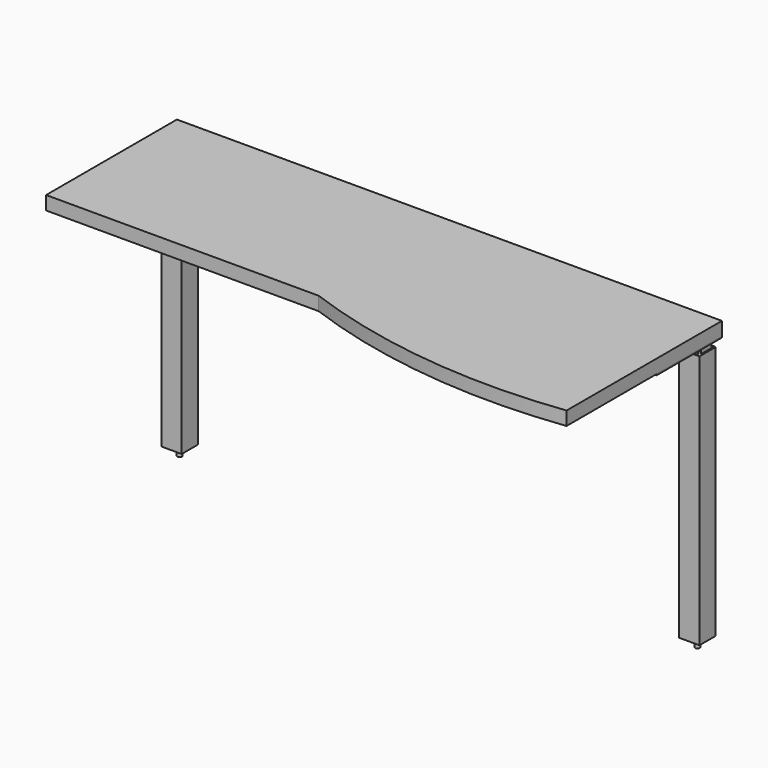
from build123d import *

# Parameters (mm, degrees)
F1_DEPTH = 38.1
F2_R     = 3.175
F2_W     = 57.0786401749
F2_H     = 56.9417057037
F2_R_2   = 6.35
F3_DEPTH = 3.175
F4_DEPTH = 685.8
F5_START = 25.4
F5_DEPTH = 25.4
F6_START = 25.4
F6_DEPTH = 711.2
F7_START = 6.35
F7_DEPTH = 755.65


with BuildPart() as f1:
    # F0 (on Top) → F1 (new body)
    with BuildSketch(Plane.XY):
        with BuildLine():
            Line((762, -250.8953552246), (762, 0))
            Line((762, 0), (762, 228.6))
            Line((762, 228.6), (0, 228.6))
            Line((0, 228.6), (-762, 228.6))
            Line((-762, 228.6), (-762, 0))
            Line((-762, 0), (-762, -228.6))
            Line((-762, -228.6), (0, -228.6))
            ThreePointArc((0, -228.6), (375.8490807179, -317.246080689), (762, -314.3953552246))
            Line((762, -314.3953552246), (762, -250.8953552246))
        make_face()
    extrude(amount=-F1_DEPTH)


with BuildPart() as f3:
    # F2 (on face) → F3 (new body)
    with BuildSketch(Plane(origin=(0, 0, -38.1), x_dir=(1, 0, 0), z_dir=(0, 0, -1))):
        Polygon((-762, -152.4), (-762, -228.6), (-685.8, -228.6), (-533.4, -228.6), (-533.4, -203.2), (-685.8, -203.2), (-685.8, -152.4), (-736.6, -152.4), (-736.6, 0), (-762, 0), align=None)
        with Locations((-647.7, -215.9)):
            Circle(F2_R, mode=Mode.SUBTRACT)
        with Locations((-609.6, -215.9)):
            Circle(F2_R, mode=Mode.SUBTRACT)
        with Locations((-723.9, -190.5)):
            Rectangle(F2_W, F2_H, mode=Mode.SUBTRACT)
        with Locations((-571.5, -215.9)):
            Circle(F2_R, mode=Mode.SUBTRACT)
        with Locations((-749.3, -114.3)):
            Circle(F2_R, mode=Mode.SUBTRACT)
        with Locations((-749.3, -76.2)):
            Circle(F2_R, mode=Mode.SUBTRACT)
        with Locations((-749.3, -38.1)):
            Circle(F2_R, mode=Mode.SUBTRACT)
        with Locations((-723.9, -190.5)):
            Rectangle(F2_W, F2_H)
        Polygon((-748.4057545662, -166.1619693041), (-745.25012113, -166.1619693041), (-699.3942454338, -166.1619693041), (-699.3942454338, -208.2879563526), (-699.3942454338, -214.8380306959), (-702.5608834128, -214.8380306959), (-748.4057545662, -214.8380306959), (-748.4057545662, -172.5196880927), align=None, mode=Mode.SUBTRACT)
        Polygon((-742.95, -209.55), (-742.95, -177.5557692308), (-746.125, -174.625), (-746.125, -212.725), (-704.85, -212.725), (-708.2895833333, -209.55), align=None)
        Polygon((-701.675, -206.1927169561), (-704.85, -203.275969498), (-704.85, -209.55), (-708.2895833333, -209.55), (-704.85, -212.725), (-701.675, -212.725), align=None)
        Polygon((-746.125, -168.275), (-742.95, -168.275), (-745.25012113, -166.1619693041), (-748.4057545662, -166.1619693041), (-748.4057545662, -172.5196880927), (-746.125, -174.625), align=None)
        Polygon((-746.125, -212.725), (-746.125, -174.625), (-748.4057545662, -172.5196880927), (-748.4057545662, -214.8380306959), (-702.5608834128, -214.8380306959), (-704.85, -212.725), align=None)
        with BuildLine():
            Line((-738.0940227608, -182.0382097593), (-742.95, -177.5557692308))
            Line((-742.95, -177.5557692308), (-742.95, -209.55))
            Line((-742.95, -209.55), (-708.2895833333, -209.55))
            Line((-708.2895833333, -209.55), (-714.3315363447, -203.9728126049))
            ThreePointArc((-714.3315363447, -203.9728126049), (-735.1085079185, -202.642550245), (-738.0940227608, -182.0382097593))
        make_face()
        with BuildLine():
            Line((-739.4938814486, -171.45), (-742.95, -171.45))
            Line((-742.95, -171.45), (-742.95, -177.5557692308))
            Line((-742.95, -177.5557692308), (-738.0940227608, -182.0382097593))
            ThreePointArc((-738.0940227608, -182.0382097593), (-735.1085079185, -202.642550245), (-714.3315363447, -203.9728126049))
            Line((-714.3315363447, -203.9728126049), (-708.2895833333, -209.55))
            Line((-708.2895833333, -209.55), (-704.85, -209.55))
            Line((-704.85, -209.55), (-704.85, -203.275969498))
            Line((-704.85, -203.275969498), (-709.6497025066, -198.866671833))
            ThreePointArc((-709.6497025066, -198.866671833), (-712.7205420695, -178.3306985989), (-733.4427339264, -177.0089509147))
            Line((-733.4427339264, -177.0089509147), (-739.4938814486, -171.45))
        make_face()
        with Locations((-723.9, -190.5)):
            Circle(F2_R_2, mode=Mode.SUBTRACT)
        with BuildLine():
            Line((-704.85, -171.45), (-739.4938814486, -171.45))
            Line((-739.4938814486, -171.45), (-733.4427339264, -177.0089509147))
            ThreePointArc((-733.4427339264, -177.0089509147), (-712.7205420695, -178.3306985989), (-709.6497025066, -198.866671833))
            Line((-709.6497025066, -198.866671833), (-704.85, -203.275969498))
            Line((-704.85, -203.275969498), (-704.85, -171.45))
        make_face()
        Polygon((-742.95, -177.5557692308), (-742.95, -171.45), (-739.4938814486, -171.45), (-742.95, -168.275), (-746.125, -168.275), (-746.125, -174.625), align=None)
        Polygon((-742.95, -168.275), (-739.4938814486, -171.45), (-704.85, -171.45), (-704.85, -203.275969498), (-701.675, -206.1927169561), (-701.675, -168.275), align=None)
        Polygon((-745.25012113, -166.1619693041), (-742.95, -168.275), (-701.675, -168.275), (-701.675, -206.1927169561), (-699.3942454338, -208.2879563526), (-699.3942454338, -166.1619693041), align=None)
        with Locations((-723.9, -190.5)):
            Circle(F2_R_2)
    extrude(amount=F3_DEPTH)

    # F2 (on face) → F4 (join)
    with BuildSketch(Plane(origin=(0, 0, -38.1), x_dir=(1, 0, 0), z_dir=(0, 0, -1))):
        Polygon((-742.95, -209.55), (-742.95, -177.5557692308), (-746.125, -174.625), (-746.125, -212.725), (-704.85, -212.725), (-708.2895833333, -209.55), align=None)
        Polygon((-742.95, -168.275), (-739.4938814486, -171.45), (-704.85, -171.45), (-704.85, -203.275969498), (-701.675, -206.1927169561), (-701.675, -168.275), align=None)
    extrude(amount=F4_DEPTH)


with BuildPart() as f3b:
    # F2 (on face) → F3, piece 2 (new body)
    with BuildSketch(Plane(origin=(0, 0, -38.1), x_dir=(1, 0, 0), z_dir=(0, 0, -1))):
        Polygon((533.4, -203.2), (533.4, -228.6), (685.8, -228.6), (762, -228.6), (762, -152.4), (762, 0), (736.6, 0), (736.6, -152.4), (685.8, -152.4), (685.8, -203.2), align=None)
        with Locations((609.6, -215.9)):
            Circle(F2_R, mode=Mode.SUBTRACT)
        with Locations((647.7, -215.9)):
            Circle(F2_R, mode=Mode.SUBTRACT)
        with Locations((723.9, -190.5)):
            Rectangle(F2_W, F2_H, mode=Mode.SUBTRACT)
        with Locations((749.3, -114.3)):
            Circle(F2_R, mode=Mode.SUBTRACT)
        with Locations((749.3, -76.2)):
            Circle(F2_R, mode=Mode.SUBTRACT)
        with Locations((749.3, -38.1)):
            Circle(F2_R, mode=Mode.SUBTRACT)
        with Locations((723.9, -190.5)):
            Rectangle(F2_W, F2_H)
        Polygon((748.4057545662, -166.1619693041), (748.4057545662, -172.5196880927), (748.4057545662, -214.8380306959), (702.5608834128, -214.8380306959), (699.3942454338, -214.8380306959), (699.3942454338, -208.2879563526), (699.3942454338, -166.1619693041), (745.25012113, -166.1619693041), align=None, mode=Mode.SUBTRACT)
        with BuildLine():
            Line((742.95, -177.5557692308), (746.125, -174.625))
            Line((746.125, -174.625), (748.4057545662, -172.5196880927))
            Line((748.4057545662, -172.5196880927), (748.4057545662, -166.1619693041))
            Line((748.4057545662, -166.1619693041), (745.25012113, -166.1619693041))
            Line((745.25012113, -166.1619693041), (742.95, -168.275))
            Line((742.95, -168.275), (739.4938814486, -171.45))
            Line((739.4938814486, -171.45), (733.4427339264, -177.0089509147))
            ThreePointArc((733.4427339264, -177.0089509147), (712.7205420695, -178.3306985989), (709.6497025066, -198.866671833))
            Line((709.6497025066, -198.866671833), (704.85, -203.275969498))
            Line((704.85, -203.275969498), (701.675, -206.1927169561))
            Line((701.675, -206.1927169561), (699.3942454338, -208.2879563526))
            Line((699.3942454338, -208.2879563526), (699.3942454338, -214.8380306959))
            Line((699.3942454338, -214.8380306959), (702.5608834128, -214.8380306959))
            Line((702.5608834128, -214.8380306959), (704.85, -212.725))
            Line((704.85, -212.725), (708.2895833333, -209.55))
            Line((708.2895833333, -209.55), (714.3315363447, -203.9728126049))
            ThreePointArc((714.3315363447, -203.9728126049), (735.1085079185, -202.642550245), (738.0940227608, -182.0382097593))
            Line((738.0940227608, -182.0382097593), (742.95, -177.5557692308))
        make_face()
        with Locations((723.9, -190.5)):
            Circle(F2_R_2, mode=Mode.SUBTRACT)
        with BuildLine():
            Line((742.95, -209.55), (742.95, -177.5557692308))
            Line((742.95, -177.5557692308), (738.0940227608, -182.0382097593))
            ThreePointArc((738.0940227608, -182.0382097593), (735.1085079185, -202.642550245), (714.3315363447, -203.9728126049))
            Line((714.3315363447, -203.9728126049), (708.2895833333, -209.55))
            Line((708.2895833333, -209.55), (742.95, -209.55))
        make_face()
        with BuildLine():
            Line((733.4427339264, -177.0089509147), (739.4938814486, -171.45))
            Line((739.4938814486, -171.45), (704.85, -171.45))
            Line((704.85, -171.45), (704.85, -203.275969498))
            Line((704.85, -203.275969498), (709.6497025066, -198.866671833))
            ThreePointArc((709.6497025066, -198.866671833), (712.7205420695, -178.3306985989), (733.4427339264, -177.0089509147))
        make_face()
        Polygon((746.125, -212.725), (746.125, -174.625), (742.95, -177.5557692308), (742.95, -209.55), (708.2895833333, -209.55), (704.85, -212.725), align=None)
        Polygon((739.4938814486, -171.45), (742.95, -168.275), (701.675, -168.275), (701.675, -206.1927169561), (704.85, -203.275969498), (704.85, -171.45), align=None)
        Polygon((748.4057545662, -172.5196880927), (746.125, -174.625), (746.125, -212.725), (704.85, -212.725), (702.5608834128, -214.8380306959), (748.4057545662, -214.8380306959), align=None)
        Polygon((742.95, -168.275), (745.25012113, -166.1619693041), (699.3942454338, -166.1619693041), (699.3942454338, -208.2879563526), (701.675, -206.1927169561), (701.675, -168.275), align=None)
        with Locations((723.9, -190.5)):
            Circle(F2_R_2)
    extrude(amount=F3_DEPTH)

    # F2 (on face) → F4, piece 2 (join)
    with BuildSketch(Plane(origin=(0, 0, -38.1), x_dir=(1, 0, 0), z_dir=(0, 0, -1))):
        Polygon((739.4938814486, -171.45), (742.95, -168.275), (701.675, -168.275), (701.675, -206.1927169561), (704.85, -203.275969498), (704.85, -171.45), align=None)
        Polygon((746.125, -212.725), (746.125, -174.625), (742.95, -177.5557692308), (742.95, -209.55), (708.2895833333, -209.55), (704.85, -212.725), align=None)
    extrude(amount=F4_DEPTH)


with BuildPart() as f5:
    # F2 (on face) → F5 (new body)
    with BuildSketch(Plane(origin=(0, 0, -38.1), x_dir=(1, 0, 0), z_dir=(0, 0, -1)).offset(F5_START)):
        with BuildLine():
            Line((-739.4938814486, -171.45), (-742.95, -171.45))
            Line((-742.95, -171.45), (-742.95, -177.5557692308))
            Line((-742.95, -177.5557692308), (-738.0940227608, -182.0382097593))
            ThreePointArc((-738.0940227608, -182.0382097593), (-735.1085079185, -202.642550245), (-714.3315363447, -203.9728126049))
            Line((-714.3315363447, -203.9728126049), (-708.2895833333, -209.55))
            Line((-708.2895833333, -209.55), (-704.85, -209.55))
            Line((-704.85, -209.55), (-704.85, -203.275969498))
            Line((-704.85, -203.275969498), (-709.6497025066, -198.866671833))
            ThreePointArc((-709.6497025066, -198.866671833), (-712.7205420695, -178.3306985989), (-733.4427339264, -177.0089509147))
            Line((-733.4427339264, -177.0089509147), (-739.4938814486, -171.45))
        make_face()
        with Locations((-723.9, -190.5)):
            Circle(F2_R_2, mode=Mode.SUBTRACT)
        Polygon((-701.675, -206.1927169561), (-704.85, -203.275969498), (-704.85, -209.55), (-708.2895833333, -209.55), (-704.85, -212.725), (-701.675, -212.725), align=None)
        Polygon((-699.3942454338, -208.2879563526), (-701.675, -206.1927169561), (-701.675, -212.725), (-704.85, -212.725), (-702.5608834128, -214.8380306959), (-699.3942454338, -214.8380306959), align=None)
        Polygon((-742.95, -177.5557692308), (-742.95, -171.45), (-739.4938814486, -171.45), (-742.95, -168.275), (-746.125, -168.275), (-746.125, -174.625), align=None)
        Polygon((-746.125, -168.275), (-742.95, -168.275), (-745.25012113, -166.1619693041), (-748.4057545662, -166.1619693041), (-748.4057545662, -172.5196880927), (-746.125, -174.625), align=None)
    extrude(amount=F5_DEPTH)

    # F2 (on face) → F6 (join)
    with BuildSketch(Plane(origin=(0, 0, -38.1), x_dir=(1, 0, 0), z_dir=(0, 0, -1)).offset(F6_START)):
        with Locations((-723.9, -190.5)):
            Rectangle(F2_W, F2_H)
        Polygon((-748.4057545662, -166.1619693041), (-745.25012113, -166.1619693041), (-699.3942454338, -166.1619693041), (-699.3942454338, -208.2879563526), (-699.3942454338, -214.8380306959), (-702.5608834128, -214.8380306959), (-748.4057545662, -214.8380306959), (-748.4057545662, -172.5196880927), align=None, mode=Mode.SUBTRACT)
    extrude(amount=F6_DEPTH)


with BuildPart() as f5b:
    # F2 (on face) → F5, piece 2 (new body)
    with BuildSketch(Plane(origin=(0, 0, -38.1), x_dir=(1, 0, 0), z_dir=(0, 0, -1)).offset(F5_START)):
        with BuildLine():
            Line((742.95, -177.5557692308), (746.125, -174.625))
            Line((746.125, -174.625), (748.4057545662, -172.5196880927))
            Line((748.4057545662, -172.5196880927), (748.4057545662, -166.1619693041))
            Line((748.4057545662, -166.1619693041), (745.25012113, -166.1619693041))
            Line((745.25012113, -166.1619693041), (742.95, -168.275))
            Line((742.95, -168.275), (739.4938814486, -171.45))
            Line((739.4938814486, -171.45), (733.4427339264, -177.0089509147))
            ThreePointArc((733.4427339264, -177.0089509147), (712.7205420695, -178.3306985989), (709.6497025066, -198.866671833))
            Line((709.6497025066, -198.866671833), (704.85, -203.275969498))
            Line((704.85, -203.275969498), (701.675, -206.1927169561))
            Line((701.675, -206.1927169561), (699.3942454338, -208.2879563526))
            Line((699.3942454338, -208.2879563526), (699.3942454338, -214.8380306959))
            Line((699.3942454338, -214.8380306959), (702.5608834128, -214.8380306959))
            Line((702.5608834128, -214.8380306959), (704.85, -212.725))
            Line((704.85, -212.725), (708.2895833333, -209.55))
            Line((708.2895833333, -209.55), (714.3315363447, -203.9728126049))
            ThreePointArc((714.3315363447, -203.9728126049), (735.1085079185, -202.642550245), (738.0940227608, -182.0382097593))
            Line((738.0940227608, -182.0382097593), (742.95, -177.5557692308))
        make_face()
        with Locations((723.9, -190.5)):
            Circle(F2_R_2, mode=Mode.SUBTRACT)
    extrude(amount=F5_DEPTH)

    # F2 (on face) → F6, piece 2 (join)
    with BuildSketch(Plane(origin=(0, 0, -38.1), x_dir=(1, 0, 0), z_dir=(0, 0, -1)).offset(F6_START)):
        with Locations((723.9, -190.5)):
            Rectangle(F2_W, F2_H)
        Polygon((748.4057545662, -166.1619693041), (748.4057545662, -172.5196880927), (748.4057545662, -214.8380306959), (702.5608834128, -214.8380306959), (699.3942454338, -214.8380306959), (699.3942454338, -208.2879563526), (699.3942454338, -166.1619693041), (745.25012113, -166.1619693041), align=None, mode=Mode.SUBTRACT)
    extrude(amount=F6_DEPTH)


with BuildPart() as f7:
    # F2 (on face) → F7 (new body)
    with BuildSketch(Plane(origin=(0, 0, -38.1), x_dir=(1, 0, 0), z_dir=(0, 0, -1)).offset(F7_START)):
        with Locations((-723.9, -190.5)):
            Circle(F2_R_2)
    extrude(amount=F7_DEPTH)


with BuildPart() as f7b:
    # F2 (on face) → F7, piece 2 (new body)
    with BuildSketch(Plane(origin=(0, 0, -38.1), x_dir=(1, 0, 0), z_dir=(0, 0, -1)).offset(F7_START)):
        with Locations((723.9, -190.5)):
            Circle(F2_R_2)
    extrude(amount=F7_DEPTH)


solid = Compound([f1.part, f3.part, f3b.part, f5.part, f5b.part, f7.part, f7b.part])
